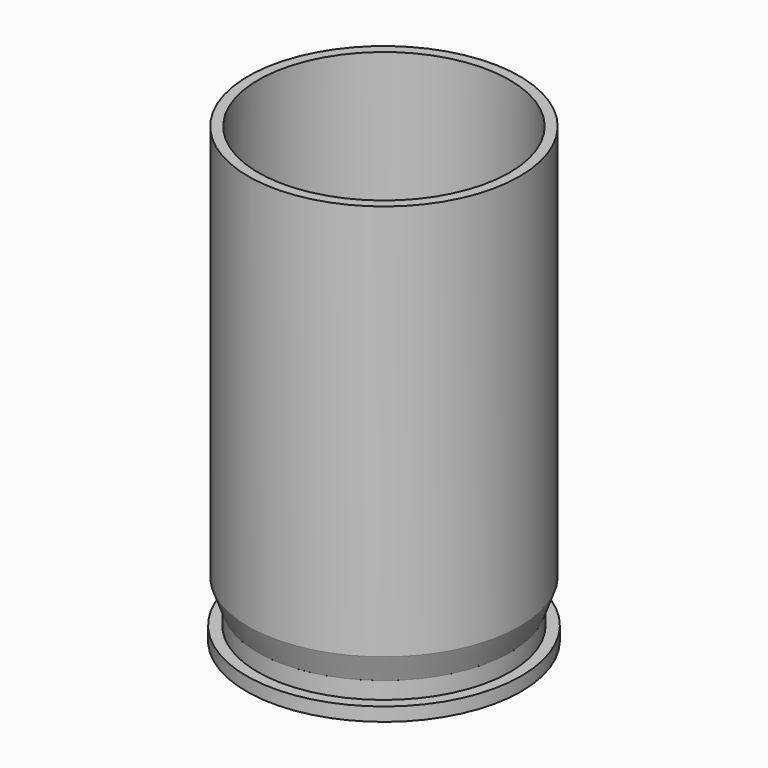
from build123d import *

# Parameters (mm, degrees)
F0_R     = 20
F0_R_2   = 18.5078276758
F1_DEPTH = 63.5
F3_R     = 18.6165604835
F3_R_2   = 17.2832490894
F4_DEPTH = 1.27
F6_R     = 20.25
F7_DEPTH = 2


# Not quite as in the source:
# - a fillet or chamfer that OpenCascade refuses, or shapes differently, is made with other operations: its cross-section is extruded or revolved along the edge and cut away or added


with BuildPart() as f1:
    # F0 (on Top) → F1 (new body)
    with BuildSketch(Plane.XY):
        Circle(F0_R)
        Circle(F0_R_2, mode=Mode.SUBTRACT)
    extrude(amount=F1_DEPTH)

    # F2: chamfer of 5.08 x 1.8489687901 on 1 edges, made by hand

    # F2_s1 → F2_t2 (revolve, cut)
    with BuildSketch(Plane.XZ):
        Polygon((20, 5.08), (18.1510312099, 0), (20, 0), align=None)
    revolve(axis=Axis((0, 0, 0), (0, 0, 1)), mode=Mode.SUBTRACT)

    # F3 (on Top) → F4 (join, symmetric)
    with BuildSketch(Plane.XY):
        Circle(F3_R)
        Circle(F3_R_2, mode=Mode.SUBTRACT)
    extrude(amount=F4_DEPTH, both=True)

    # F6 (on offset) → F7 (join)
    with BuildSketch(Plane.XY.offset(-1.2446)):
        Circle(F6_R)
    extrude(amount=-F7_DEPTH)


solid = f1.part
